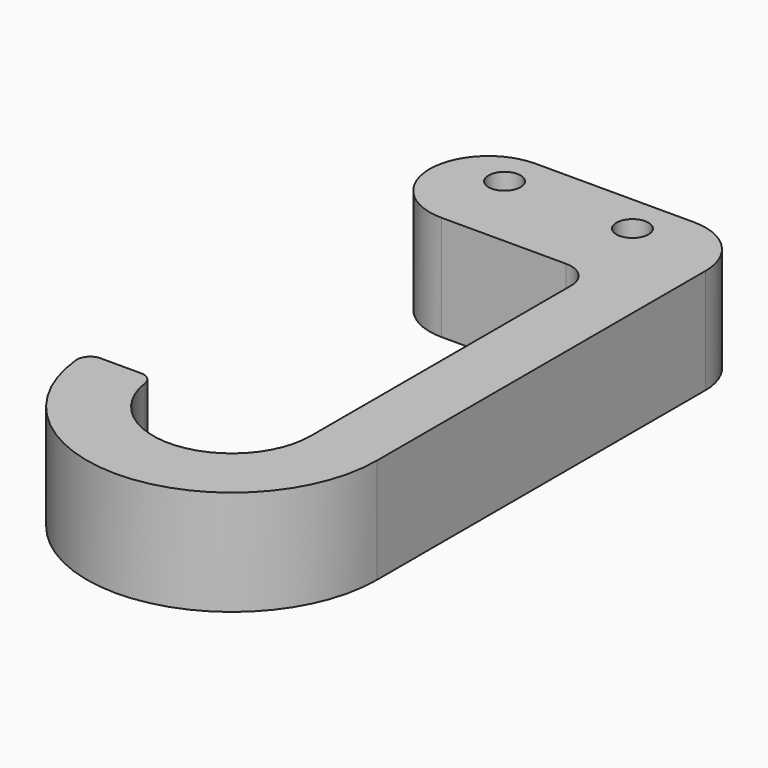
from build123d import *

# Parameters (mm, degrees)
F0_R     = 1.9332973568
F1_DEPTH = 6.35


# Not quite as in the source:
# - a feature names something its author has since deleted; it is built from what else it names


with BuildPart() as f1:
    # F0 (on Top) → F1 (new body, symmetric)
    with BuildSketch(Plane.XY):
        with BuildLine():
            ThreePointArc((-15.8833512398, 0), (-17.0603794097, -0.5222484159), (-17.4629810004, -1.7453799214))
            ThreePointArc((-17.4629810004, -1.7453799214), (0.8737735944, -17.5282222771), (17.5499873644, 0))
            Line((17.5499873644, 0), (17.5499873644, 49.6334969772))
            ThreePointArc((17.5499873644, 49.6334969772), (15.4732281229, 54.6472373039), (10.4594877962, 56.7239965454))
            Line((10.4594877962, 56.7239965454), (-8.711161666, 56.7239965454))
            ThreePointArc((-8.711161666, 56.7239965454), (-14.3252844017, 53.9644102799), (-15.5694312717, 47.8336852809))
            ThreePointArc((-15.5694312717, 47.8336852809), (-13.0420749687, 44.0193742416), (-8.711161666, 42.5429974091))
            Line((-8.711161666, 42.5429974091), (6.35, 42.5429974091))
            ThreePointArc((6.35, 42.5429974091), (8.5950640303, 41.6130614393), (9.525, 39.3679974091))
            Line((9.525, 39.3679974091), (9.525, 0))
            ThreePointArc((9.525, 0), (0.6821084333, -9.5005448836), (-9.4273051098, -1.3607142857))
            ThreePointArc((-9.4273051098, -1.3607142857), (-9.9592599258, -0.3874627982), (-10.9985226281, 0))
            Line((-10.9985226281, 0), (-15.8833512398, 0))
        make_face()
        with Locations((-8.711161666, 52.084082889)):
            Circle(F0_R, mode=Mode.SUBTRACT)
        with Locations((6.7552171887, 52.084082889)):
            Circle(F0_R, mode=Mode.SUBTRACT)
    extrude(amount=F1_DEPTH, both=True)


solid = f1.part
